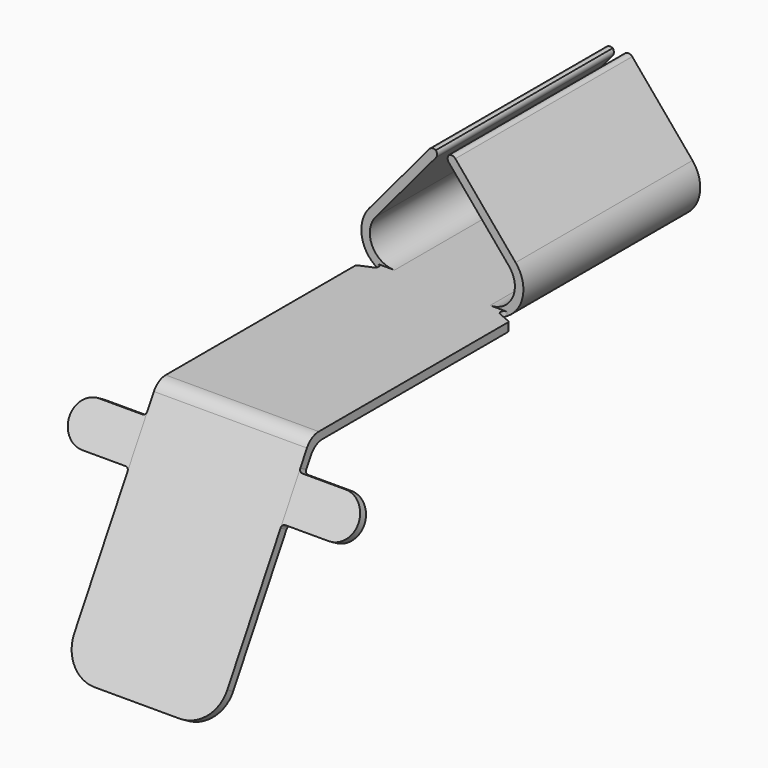
from build123d import *

# Parameters (mm, degrees)
F1_DEPTH      = 13
F3_W          = 5.624003956
F3_H          = 13
F4_DEPTH      = 0.5
F6_DEPTH      = 9
F8_W          = 1.375
F8_H          = 2.5
F9_DEPTH      = 0.5
F10_R         = 2
F11_R         = 1
F12_T1_DEPTH  = 14.5
F13_T1_DEPTH  = 0.5
F13_T6_DEPTH  = 0.5
F13_S7_R      = 1.95289555
F13_T8_DEPTH  = 2
F13_T12_DEPTH = 0.5
F13_S13_R     = 1.95289555
F13_T14_DEPTH = 2


# Not quite as in the source:
# - a fillet or chamfer that OpenCascade refuses, or shapes differently, is made with other operations: its cross-section is extruded or revolved along the edge and cut away or added


with BuildPart() as f1:
    # F0 (on Front) → F1 (new body)
    with BuildSketch(Plane.XZ):
        with BuildLine():
            Line((-0.1891016816, 7.3390506263), (-0.5721239031, 7.6604444312))
            Line((-0.5721239031, 7.6604444312), (-4.3080067621, 3.2081926126))
            ThreePointArc((-4.3080067621, 3.2081926126), (-4.5819264222, 1.1275662273), (-2.812001978, 0))
            Line((-2.812001978, 0), (0, 0))
            Line((0, 0), (0, 0.5))
            Line((0, 0.5), (-2.812001978, 0.5))
            ThreePointArc((-2.812001978, 0.5), (-4.1287725287, 1.3388753582), (-3.9249845405, 2.8867988077))
            Line((-3.9249845405, 2.8867988077), (-0.1891016816, 7.3390506263))
        make_face()
        with BuildLine():
            Line((0, 0.5), (0, 0))
            Line((0, 0), (2.812001978, 0))
            ThreePointArc((2.812001978, 0), (4.5819264222, 1.1275662273), (4.3080067621, 3.2081926126))
            Line((4.3080067621, 3.2081926126), (0.5721239031, 7.6604444312))
            Line((0.5721239031, 7.6604444312), (0.1891016816, 7.3390506263))
            Line((0.1891016816, 7.3390506263), (3.9249845405, 2.8867988077))
            ThreePointArc((3.9249845405, 2.8867988077), (4.1287725287, 1.3388753582), (2.812001978, 0.5))
            Line((2.812001978, 0.5), (0, 0.5))
        make_face()
    extrude(amount=-F1_DEPTH)

    # F3 (on offset) → F4 (join, through all)
    with BuildSketch(Plane(origin=(0, 0, 0), x_dir=(1, 0, 0), z_dir=(0, 0, -1))):
        with Locations((0, -6.5)):
            Rectangle(F3_W, F3_H)
        with BuildLine():
            Line((-2.812001978, 0), (2.812001978, 0))
            Line((2.812001978, 0), (4.4072171914, 0.6821090398))
            ThreePointArc((4.4072171914, 0.6821090398), (4.4747132661, 0.7384715991), (4.5, 0.8226917824))
            Line((4.5, 0.8226917824), (4.5, 15))
            Line((4.5, 15), (-4.5, 15))
            Line((-4.5, 15), (-4.5, 0.8226917824))
            ThreePointArc((-4.5, 0.8226917824), (-4.4747132661, 0.7384715991), (-4.4072171914, 0.6821090398))
            Line((-4.4072171914, 0.6821090398), (-2.812001978, 0))
        make_face()
    extrude(amount=-F4_DEPTH)

    # F5 (on face) → F6 (join, through all)
    with BuildSketch(Plane.YZ.offset(4.5)):
        Polygon((-22.4330127019, -11.874355653), (-22, -12.124355653), (-15, 0), (-15, 0.5), (-15.2886751346, 0.5), align=None)
    extrude(amount=-F6_DEPTH)

    # F8 (on offset) → F9 (join, through all)
    with BuildSketch(Plane(origin=(0, -11.6830127019, 6.7451905284), x_dir=(1, 0, 0), z_dir=(0, -0.8660254038, 0.5))):
        with Locations((-5.1875, -10.2113248654)):
            Rectangle(F8_W, F8_H)
        with BuildLine():
            Line((-5.875, -11.4613248654), (-5.875, -8.9613248654))
            Line((-5.875, -8.9613248654), (-7.25, -8.9613248654))
            ThreePointArc((-7.25, -8.9613248654), (-8.5, -10.2113248654), (-7.25, -11.4613248654))
            Line((-7.25, -11.4613248654), (-5.875, -11.4613248654))
        make_face()
        Polygon((4.5, -7.2113248654), (-4.5, -7.2113248654), (-4.5, -8.9613248654), (-4.5, -11.4613248654), (-4.5, -13.2113248654), (4.5, -13.2113248654), (4.5, -11.4613248654), (5.875, -11.4613248654), (5.875, -8.9613248654), (4.5, -8.9613248654), align=None)
        with BuildLine():
            Line((7.25, -8.9613248654), (5.875, -8.9613248654))
            Line((5.875, -8.9613248654), (5.875, -11.4613248654))
            Line((5.875, -11.4613248654), (7.25, -11.4613248654))
            ThreePointArc((7.25, -11.4613248654), (8.5, -10.2113248654), (7.25, -8.9613248654))
        make_face()
    extrude(amount=-F9_DEPTH)

    # F10
    f10_edges = [f1.edges().sort_by_distance(p)[0] for p in [
        (4.5, -22.216506, -11.999356),
        (-4.5, -22.216506, -11.999356),
    ]]
    fillet(f10_edges, radius=F10_R)

    # F11
    f11_edges = [f1.edges().sort_by_distance(p)[0] for p in [
        (0, -15.288675, 0.5),
        (0, -15, 0),
    ]]
    fillet(f11_edges, radius=F11_R)

    # F12: fillet of radius 0.3 on 4 edges, made by hand

    # F12_s2 → F12_t1 (cut)
    with BuildSketch(Plane.XZ.offset(-13.75)):
        with BuildLine():
            ThreePointArc((0.4189150145, 7.5318869093), (0.312892888, 7.3282202991), (0.3819379645, 7.1092372934))
            Line((0.3819379645, 7.1092372934), (0.1891016816, 7.3390506263))
            Line((0.1891016816, 7.3390506263), (0.4189150145, 7.5318869093))
        make_face()
        with BuildLine():
            ThreePointArc((-0.3819379645, 7.1092372934), (-0.312892888, 7.3282202991), (-0.4189150145, 7.5318869093))
            Line((-0.4189150145, 7.5318869093), (-0.1891016816, 7.3390506263))
            Line((-0.1891016816, 7.3390506263), (-0.3819379645, 7.1092372934))
        make_face()
        with BuildLine():
            ThreePointArc((0.764960186, 7.4306310983), (0.5612935759, 7.5366532248), (0.3423105702, 7.4676081483))
            Line((0.3423105702, 7.4676081483), (0.5721239031, 7.6604444312))
            Line((0.5721239031, 7.6604444312), (0.764960186, 7.4306310983))
        make_face()
        with BuildLine():
            ThreePointArc((-0.3423105702, 7.4676081483), (-0.5612935759, 7.5366532248), (-0.764960186, 7.4306310983))
            Line((-0.764960186, 7.4306310983), (-0.5721239031, 7.6604444312))
            Line((-0.5721239031, 7.6604444312), (-0.3423105702, 7.4676081483))
        make_face()
    extrude(amount=F12_T1_DEPTH, mode=Mode.SUBTRACT)

    # F13: fillet of radius 0.2 on 6 edges, made by hand

    # F13_s2 → F13_t1 (join)
    with BuildSketch(Plane(origin=(0, -11.6830127019, 6.7451905284), x_dir=(1, 0, 0), z_dir=(0, 0.8660254038, -0.5))):
        with BuildLine():
            ThreePointArc((-4.5, 8.7613248654), (-4.5585786438, 8.9027462216), (-4.7, 8.9613248654))
            Line((-4.7, 8.9613248654), (-4.5, 8.9613248654))
            Line((-4.5, 8.9613248654), (-4.5, 8.7613248654))
        make_face()
        with BuildLine():
            ThreePointArc((-4.7, 11.4613248654), (-4.5585786438, 11.5199035092), (-4.5, 11.6613248654))
            Line((-4.5, 11.6613248654), (-4.5, 11.4613248654))
            Line((-4.5, 11.4613248654), (-4.7, 11.4613248654))
        make_face()
        with BuildLine():
            ThreePointArc((4.5, 8.7613248654), (4.5585786438, 8.9027462216), (4.7, 8.9613248654))
            Line((4.7, 8.9613248654), (4.5, 8.9613248654))
            Line((4.5, 8.9613248654), (4.5, 8.7613248654))
        make_face()
        with BuildLine():
            ThreePointArc((4.7, 11.4613248654), (4.5585786438, 11.5199035092), (4.5, 11.6613248654))
            Line((4.5, 11.6613248654), (4.5, 11.4613248654))
            Line((4.5, 11.4613248654), (4.7, 11.4613248654))
        make_face()
    extrude(amount=F13_T1_DEPTH)


with BuildPart() as f13_tool4:
    # F13_s5 → F13_t6 (new body)
    with BuildSketch(Plane.XY):
        with BuildLine():
            ThreePointArc((3.7097957982, -0.3838938316), (3.5924961377, -0.159867509), (3.7884282258, 0))
            Line((3.7884282258, 0), (2.812001978, 0))
            Line((2.812001978, 0), (3.7097957982, -0.3838938316))
        make_face()
    extrude(amount=F13_T6_DEPTH)

    # F13_s7 → F13_t8 (intersect, symmetric)
    with BuildSketch(Plane.XZ.offset(0.2)):
        with Locations((2.812001978, 1.95289555)):
            Circle(F13_S7_R)
    extrude(amount=F13_T8_DEPTH, both=True, mode=Mode.INTERSECT)


with BuildPart() as f1_1:
    add(f1.part)

    # F13_t3: union F13_tool4
    add(f13_tool4.part)


with BuildPart() as f13_tool10:
    # F13_s11 → F13_t12 (new body)
    with BuildSketch(Plane.XY):
        with BuildLine():
            ThreePointArc((-3.7097957982, -0.3838938316), (-3.5924961377, -0.159867509), (-3.7884282258, 0))
            Line((-3.7884282258, 0), (-2.812001978, 0))
            Line((-2.812001978, 0), (-3.7097957982, -0.3838938316))
        make_face()
    extrude(amount=F13_T12_DEPTH)

    # F13_s13 → F13_t14 (intersect, symmetric)
    with BuildSketch(Plane.XZ.offset(0.2)):
        with Locations((-2.812001978, 1.95289555)):
            Circle(F13_S13_R)
    extrude(amount=F13_T14_DEPTH, both=True, mode=Mode.INTERSECT)


with BuildPart() as f1_2:
    add(f1_1.part)

    # F13_t9: union F13_tool10
    add(f13_tool10.part)


solid = f1_2.part
